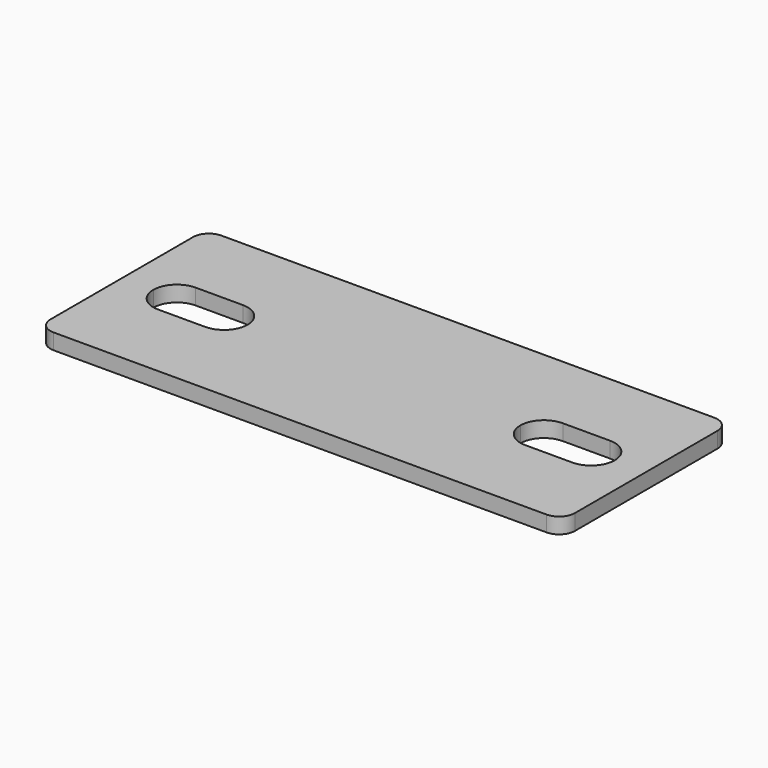
from build123d import *

# Parameters (mm, degrees)
F0_W     = 100
F0_H     = 40
F1_DEPTH = 3
F2_R     = 3
F3_W     = 18
F3_H     = 9
F4_DEPTH = 25
F5_R     = 4.49999
F6_R     = 4.49999


# Not quite as in the source:
# - a fillet or chamfer is up to 0.001 mm smaller than in the source, because OpenCascade refuses the exact size


with BuildPart() as f1:
    # F0 (on Top) → F1 (new body)
    with BuildSketch(Plane.XY):
        Rectangle(F0_W, F0_H)
    extrude(amount=F1_DEPTH)

    # F2
    f2_edges = [f1.edges().sort_by_distance(p)[0] for p in [
        (50, -20, 1.5),
        (50, 20, 1.5),
        (-50, -20, 1.5),
        (-50, 20, 1.5),
    ]]
    fillet(f2_edges, radius=F2_R)

    # F3 (on face) → F4 (cut)
    with BuildSketch(Plane.XY.offset(3)):
        with Locations((-35, 0)):
            Rectangle(F3_W, F3_H)
        with Locations((35, 0)):
            Rectangle(F3_W, F3_H)
    extrude(amount=-F4_DEPTH, mode=Mode.SUBTRACT)

    # F5 (radius 4.5 in the source; OpenCascade refuses exactly that, so slightly less here)
    f5_edges = [f1.edges().sort_by_distance(p)[0] for p in [
        (-44, 4.5, 1.5),
        (-26, 4.5, 1.5),
        (-26, -4.5, 1.5),
        (-44, -4.5, 1.5),
    ]]
    fillet(f5_edges, radius=F5_R)

    # F6 (radius 4.5 in the source; OpenCascade refuses exactly that, so slightly less here)
    f6_edges = [f1.edges().sort_by_distance(p)[0] for p in [
        (26, 4.5, 1.5),
        (44, 4.5, 1.5),
        (44, -4.5, 1.5),
        (26, -4.5, 1.5),
    ]]
    fillet(f6_edges, radius=F6_R)


solid = f1.part
